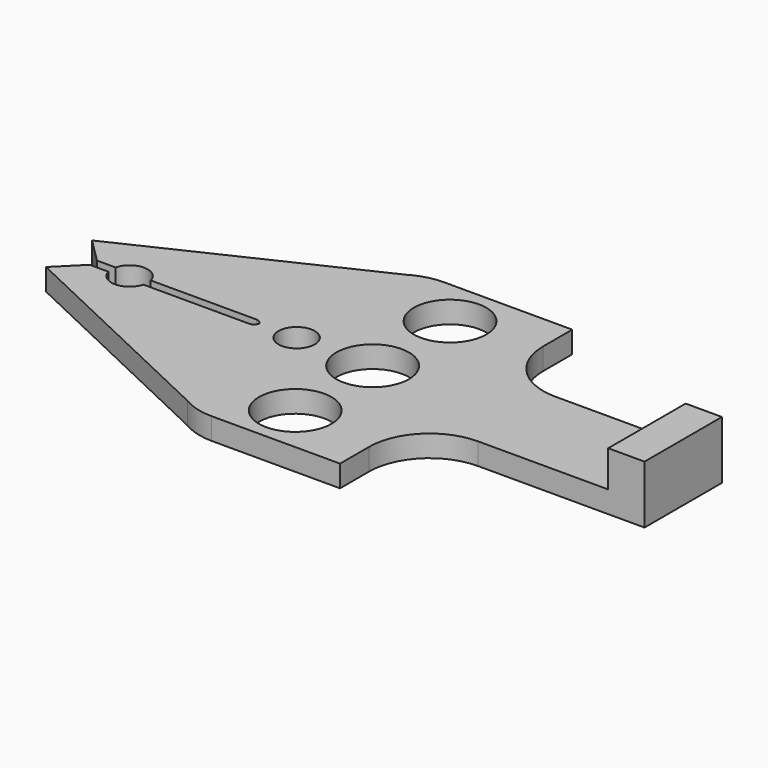
from build123d import *

# Parameters (mm, degrees)
F0_W        = 18.7768550515
F0_H        = 8
F0_W_2      = 1.2231449485
F1_DEPTH    = 1.8
F2_R        = 3
F2_R_2      = 1.5
F3_DEPTH    = 1.801
F4_W        = 3
F4_H        = 8
F5_DEPTH    = 3
F6_R        = 5
F7_T1_DEPTH = 1.8


# Not quite as in the source:
# - a fillet or chamfer that OpenCascade refuses, or shapes differently, is made with other operations: its cross-section is extruded or revolved along the edge and cut away or added


with BuildPart() as f1:
    # F0 (on Top) → F1 (new body)
    with BuildSketch(Plane.XY):
        with BuildLine():
            ThreePointArc((-1.1898192428, -11.2838109608), (0.0506537792, -11.8176267396), (1.3887392017, -12))
            Line((1.3887392017, -12), (12, -12))
            Line((12, -12), (12, -4))
            Line((12, -4), (10.7768550515, -4))
            Line((10.7768550515, -4), (10.7768550515, 4))
            Line((10.7768550515, 4), (12, 4))
            Line((12, 4), (12, 12))
            Line((12, 12), (1.3906232978, 12))
            ThreePointArc((1.3906232978, 12), (0.0508527618, 11.8171583855), (-1.1909314511, 11.2820059643))
            Line((-1.1909314511, 11.2820059643), (-19.9959281202, 2.3695112828))
            Line((-19.9959281202, 2.3695112828), (-17.9959281202, 0.3695112828))
            Line((-17.9959281202, 0.3695112828), (-16.4537748835, 0.3695112828))
            ThreePointArc((-16.4537748835, 0.3695112828), (-15, 1.5), (-13.5462251165, 0.3695112828))
            Line((-13.5462251165, 0.3695112828), (-4.2914064974, 0.3695112828))
            Line((-4.2914064974, 0.3695112828), (-4.2914064974, -0.3879051656))
            Line((-4.2914064974, -0.3879051656), (-13.5510246439, -0.3879051656))
            ThreePointArc((-13.5510246439, -0.3879051656), (-15, -1.5), (-16.4489753561, -0.3879051656))
            Line((-16.4489753561, -0.3879051656), (-17.9941705506, -0.3879051656))
            Line((-17.9941705506, -0.3879051656), (-19.9941705506, -2.3879051656))
            Line((-19.9941705506, -2.3879051656), (-1.1898192428, -11.2838109608))
        make_face()
        with Locations((21.3884275258, 0)):
            Rectangle(F0_W, F0_H)
        with Locations((11.3884275258, 0)):
            Rectangle(F0_W_2, F0_H)
    extrude(amount=F1_DEPTH)

    # F2 (on face) → F3 (cut, through all)
    with BuildSketch(Plane.XY.offset(1.8)):
        with Locations((5.0964765251, 8)):
            Circle(F2_R)
        with Locations((5.0964765251, 0)):
            Circle(F2_R)
        with Locations((5.0964765251, -8)):
            Circle(F2_R)
        with Locations((-1.1856243946, 0)):
            Circle(F2_R_2)
    extrude(amount=-F3_DEPTH, mode=Mode.SUBTRACT)

    # F4 (on face) → F5 (join)
    with BuildSketch(Plane.XY.offset(1.8)):
        with Locations((29.2768550515, 0)):
            Rectangle(F4_W, F4_H)
    extrude(amount=F5_DEPTH)

    # F6
    f6_edges = [f1.edges().sort_by_distance(p)[0] for p in [
        (12, 4, 0.9),
        (12, -4, 0.9),
    ]]
    fillet(f6_edges, radius=F6_R)

    # F7: fillet of radius 0.5 on 2 edges, made by hand

    # F7_s2 → F7_t1 (join)
    with BuildSketch(Plane.XY):
        with BuildLine():
            ThreePointArc((-4.2914064974, 0.1120948344), (-4.4378531068, -0.2414585561), (-4.7914064974, -0.3879051656))
            Line((-4.7914064974, -0.3879051656), (-4.2914064974, -0.3879051656))
            Line((-4.2914064974, -0.3879051656), (-4.2914064974, 0.1120948344))
        make_face()
        with BuildLine():
            ThreePointArc((-4.7914064974, 0.3695112828), (-4.4378531068, 0.2230646734), (-4.2914064974, -0.1304887172))
            Line((-4.2914064974, -0.1304887172), (-4.2914064974, 0.3695112828))
            Line((-4.2914064974, 0.3695112828), (-4.7914064974, 0.3695112828))
        make_face()
    extrude(amount=F7_T1_DEPTH)


solid = f1.part
